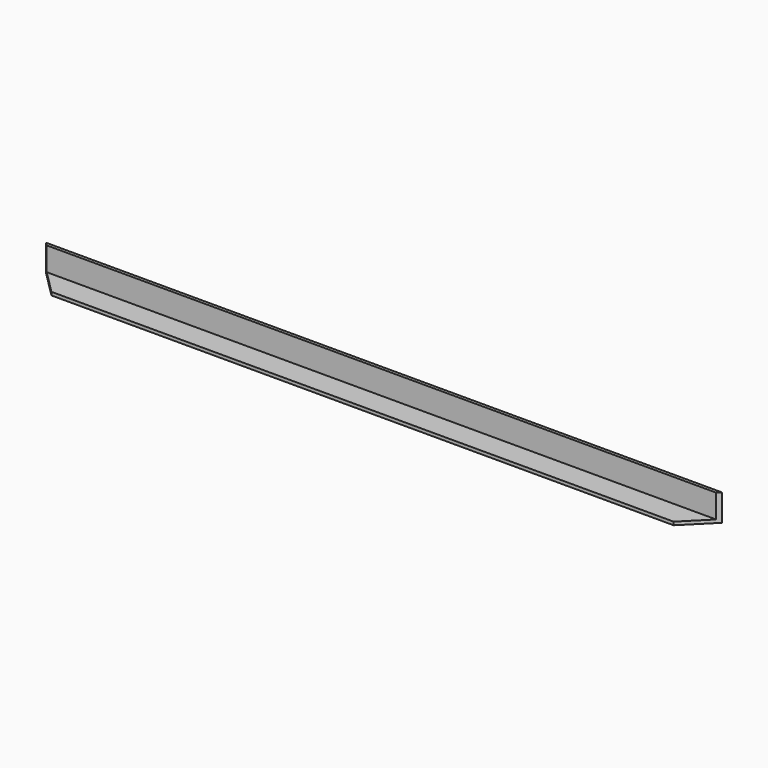
from build123d import *

# Parameters (mm, degrees)
F1_DEPTH    = 634
F2_T1_DEPTH = 47.7168298797
F4_DEPTH    = 25


# Not quite as in the source:
# - a fillet or chamfer that OpenCascade refuses, or shapes differently, is made with other operations: its cross-section is extruded or revolved along the edge and cut away or added


with BuildPart() as f1:
    # F0 (on Right) → F1 (new body)
    with BuildSketch(Plane.YZ):
        Polygon((0, 3), (0, 0), (25, 0), (25, 25), (22, 25), (22, 3), align=None)
    extrude(amount=F1_DEPTH)

    # F2: chamfer of 5 on 2 edges, made by hand

    # F2_s2 → F2_t1 (cut)
    with BuildSketch(Plane.XY.offset(-9.8584149398)):
        Polygon((629, 22), (634, 27), (634, 22), align=None)
        Polygon((5, 22), (0, 27), (0, 22), align=None)
    extrude(amount=F2_T1_DEPTH, mode=Mode.SUBTRACT)

    # F3 (on face) → F4 (cut)
    with BuildSketch(Plane.XY.offset(3)):
        Polygon((634, 22), (629, 22), (607, 0), (634, 0), align=None)
        Polygon((27, 0), (5, 22), (0, 22), (0, 0), align=None)
    extrude(amount=-F4_DEPTH, mode=Mode.SUBTRACT)


solid = f1.part
